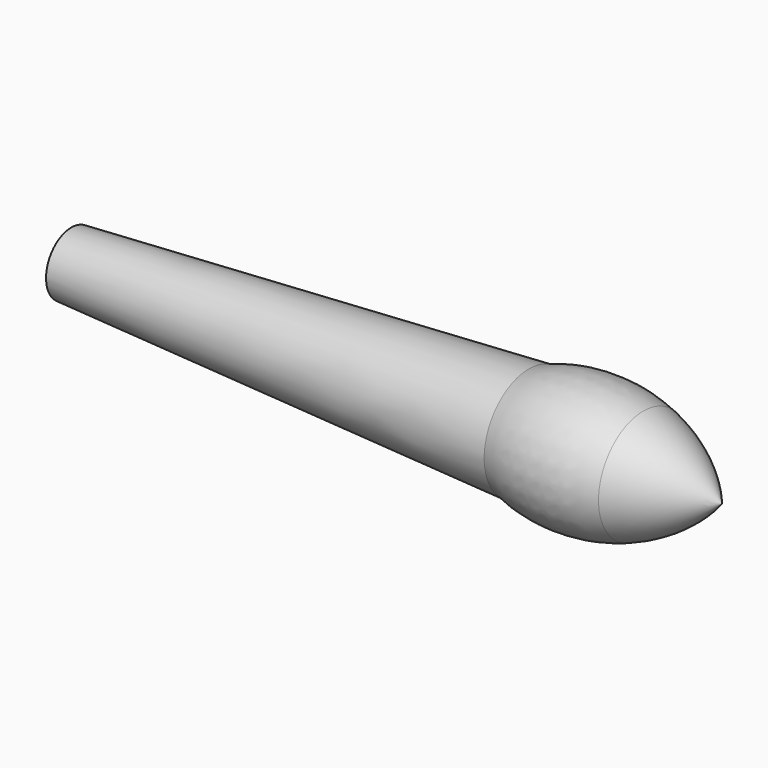
from build123d import *


# Not quite as in the source:
# - a feature names something its author has since deleted; it is built from what else it names


with BuildPart() as f1:
    # F0 (on Top) → F1 (revolve)
    with BuildSketch(Plane.XY):
        with BuildLine():
            ThreePointArc((901.9500651693, 116.8657471522), (844.7032563472, 87.2506539829), (797.971931054, 42.8610820084))
            Line((797.971931054, 42.8610820084), (1157.1030999516, 42.8610820084))
            ThreePointArc((1157.1030999516, 42.8610820084), (1110.3717746584, 87.2506539829), (1053.1249658363, 116.8657471522))
            ThreePointArc((1053.1249658363, 116.8657471522), (977.5375155028, 129.6954789984), (901.9500651693, 116.8657471522))
        make_face()
        with BuildLine():
            Line((297.0245311433, 84.7388050565), (297.0245311433, 42.8610820084))
            Line((297.0245311433, 42.8610820084), (797.971931054, 42.8610820084))
            ThreePointArc((797.971931054, 42.8610820084), (844.7032563472, 87.2506539829), (901.9500651693, 116.8657471522))
            Line((901.9500651693, 116.8657471522), (297.0245311433, 84.7388050565))
        make_face()
    revolve(axis=Axis((1412.8638155475, 42.8610820084, 0), (1, 0, 0)))


solid = f1.part
